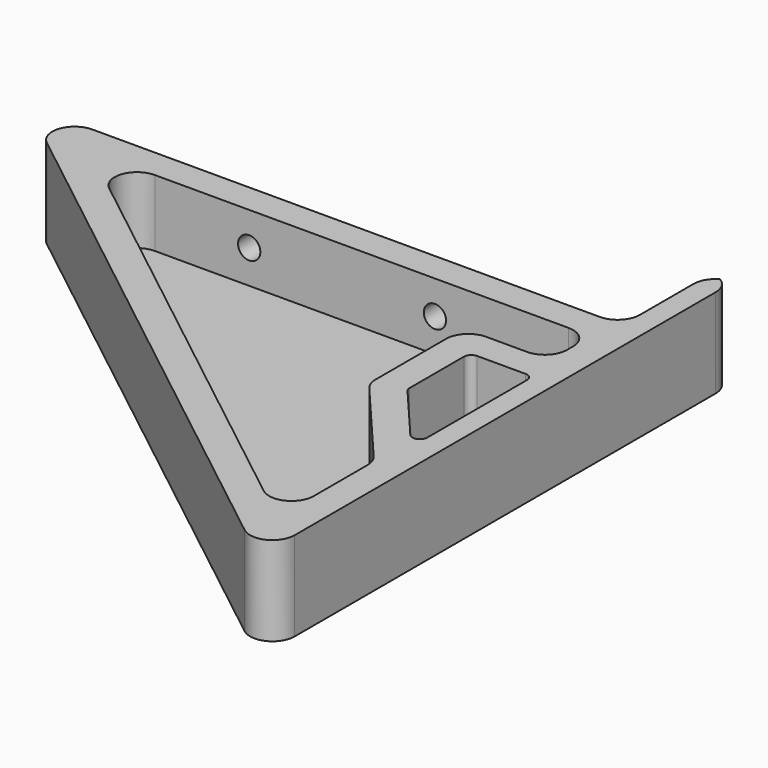
from build123d import *

# Parameters (mm, degrees)
F1_DEPTH     = 12
F3_DEPTH     = 9
F4_R         = 1.5
F5_DEPTH     = 4
F6_T1_DEPTH  = 12
F6_T3_DEPTH  = 9
F6_T5_DEPTH  = 11.7568277192
F6_T7_DEPTH  = 16.5
F6_T9_DEPTH  = 11.7568277192
F6_T11_DEPTH = 55.4822209965
F6_T13_DEPTH = 27
F6_T15_DEPTH = 42.7993296961
F7_R         = 1


# Not quite as in the source:
# - a fillet or chamfer that OpenCascade refuses, or shapes differently, is made with other operations: its cross-section is extruded or revolved along the edge and cut away or added


with BuildPart() as f1:
    # F0 (on Top) → F1 (new body)
    with BuildSketch(Plane.XY):
        Polygon((-83, 65), (0, 0), (0, 80), (-3, 80), (-3, 65), align=None)
        Polygon((-11.5, 50), (-3, 50), (-3, 29.5), (-11.5, 39.5), align=None, mode=Mode.SUBTRACT)
    extrude(amount=F1_DEPTH)

    # F2 (on face) → F3 (cut)
    with BuildSketch(Plane.XY.offset(12)):
        Polygon((-4, 54), (-4, 61), (-71.4047410676, 61), (-4, 8.2131545856), (-4, 24.5002801184), (-15.5, 38.0296918831), (-15.5, 54), align=None)
    extrude(amount=-F3_DEPTH, mode=Mode.SUBTRACT)

    # F4 (on face) → F5 (cut)
    with BuildSketch(Plane(origin=(0, 65, 0), x_dir=(-1, 0, 0), z_dir=(0, 1, 0))):
        with Locations((50, 7.5)):
            Circle(F4_R)
        with Locations((25, 7.5)):
            Circle(F4_R)
    extrude(amount=-F5_DEPTH, mode=Mode.SUBTRACT)

    # F6: fillet of radius 3 on 12 edges, made by hand

    # F6_s2 → F6_t1 (join)
    with BuildSketch(Plane.XY):
        with BuildLine():
            ThreePointArc((-6, 65), (-3.8786796564, 65.8786796564), (-3, 68))
            Line((-3, 68), (-3, 65))
            Line((-3, 65), (-6, 65))
        make_face()
    extrude(amount=F6_T1_DEPTH)

    # F6_s4 → F6_t3 (join)
    with BuildSketch(Plane.XY.offset(3)):
        with BuildLine():
            ThreePointArc((-4, 57), (-4.8786796564, 54.8786796564), (-7, 54))
            Line((-7, 54), (-4, 54))
            Line((-4, 54), (-4, 57))
        make_face()
        with BuildLine():
            ThreePointArc((-4, 58), (-4.8786796564, 60.1213203436), (-7, 61))
            Line((-7, 61), (-4, 61))
            Line((-4, 61), (-4, 58))
        make_face()
        with BuildLine():
            ThreePointArc((-8.8496919869, 12.0111061416), (-5.6864315702, 11.6758853817), (-4, 14.3730205248))
            Line((-4, 14.3730205248), (-4, 8.2131545856))
            Line((-4, 8.2131545856), (-8.8496919869, 12.0111061416))
        make_face()
        with BuildLine():
            ThreePointArc((-62.7082968683, 61), (-65.544292562, 58.9783294052), (-64.5579888552, 55.6380856168))
            Line((-64.5579888552, 55.6380856168), (-71.4047410676, 61))
            Line((-71.4047410676, 61), (-62.7082968683, 61))
        make_face()
    extrude(amount=F6_T3_DEPTH)

    # F6_s6 → F6_t5 (join)
    with BuildSketch(Plane.XY.offset(0.2431722808)):
        with BuildLine():
            ThreePointArc((-4, 23.3975490307), (-4.1842004812, 24.4325722527), (-4.7141820467, 25.340494291))
            Line((-4.7141820467, 25.340494291), (-4, 24.5002801184))
            Line((-4, 24.5002801184), (-4, 23.3975490307))
        make_face()
    extrude(amount=F6_T5_DEPTH)

    # F6_s8 → F6_t7 (cut)
    with BuildSketch(Plane.XY.offset(3)):
        with BuildLine():
            ThreePointArc((-15.5, 51), (-14.6213203436, 53.1213203436), (-12.5, 54))
            Line((-12.5, 54), (-15.5, 54))
            Line((-15.5, 54), (-15.5, 51))
        make_face()
    extrude(amount=F6_T7_DEPTH, mode=Mode.SUBTRACT)

    # F6_s10 → F6_t9 (cut)
    with BuildSketch(Plane.XY.offset(3)):
        with BuildLine():
            ThreePointArc((-14.7858179533, 37.1894777105), (-15.3157995188, 38.0973997488), (-15.5, 39.1324229708))
            Line((-15.5, 39.1324229708), (-15.5, 38.0296918831))
            Line((-15.5, 38.0296918831), (-14.7858179533, 37.1894777105))
        make_face()
    extrude(amount=F6_T9_DEPTH, mode=Mode.SUBTRACT)

    # F6_s12 → F6_t11 (cut)
    with BuildSketch(Plane.XY.offset(-21.7411104983)):
        with BuildLine():
            ThreePointArc((-76.1532477876, 59.6380856168), (-77.1395514944, 62.9783294052), (-74.3035558007, 65))
            Line((-74.3035558007, 65), (-83, 65))
            Line((-83, 65), (-76.1532477876, 59.6380856168))
        make_face()
    extrude(amount=F6_T11_DEPTH, mode=Mode.SUBTRACT)

    # F6_s14 → F6_t13 (cut)
    with BuildSketch(Plane.XY.offset(-7.5)):
        with BuildLine():
            ThreePointArc((0, 80), (-2.1213203436, 79.1213203436), (-3, 77))
            Line((-3, 77), (-3, 80))
            Line((-3, 80), (0, 80))
        make_face()
        with BuildLine():
            ThreePointArc((0, 77), (-0.8786796564, 79.1213203436), (-3, 80))
            Line((-3, 80), (0, 80))
            Line((0, 80), (0, 77))
        make_face()
    extrude(amount=F6_T13_DEPTH, mode=Mode.SUBTRACT)

    # F6_s16 → F6_t15 (cut)
    with BuildSketch(Plane.XY.offset(-15.399664848)):
        with BuildLine():
            ThreePointArc((-4.8496919869, 3.797951556), (-1.6864315702, 3.4627307961), (0, 6.1598659392))
            Line((0, 6.1598659392), (0, 0))
            Line((0, 0), (-4.8496919869, 3.797951556))
        make_face()
    extrude(amount=F6_T15_DEPTH, mode=Mode.SUBTRACT)

    # F7
    f7_edges = [f1.edges().sort_by_distance(p)[0] for p in [
        (-11.5, 50, 6),
        (-3, 50, 6),
        (-11.5, 39.5, 6),
        (-3, 29.5, 6),
    ]]
    fillet(f7_edges, radius=F7_R)


solid = f1.part
